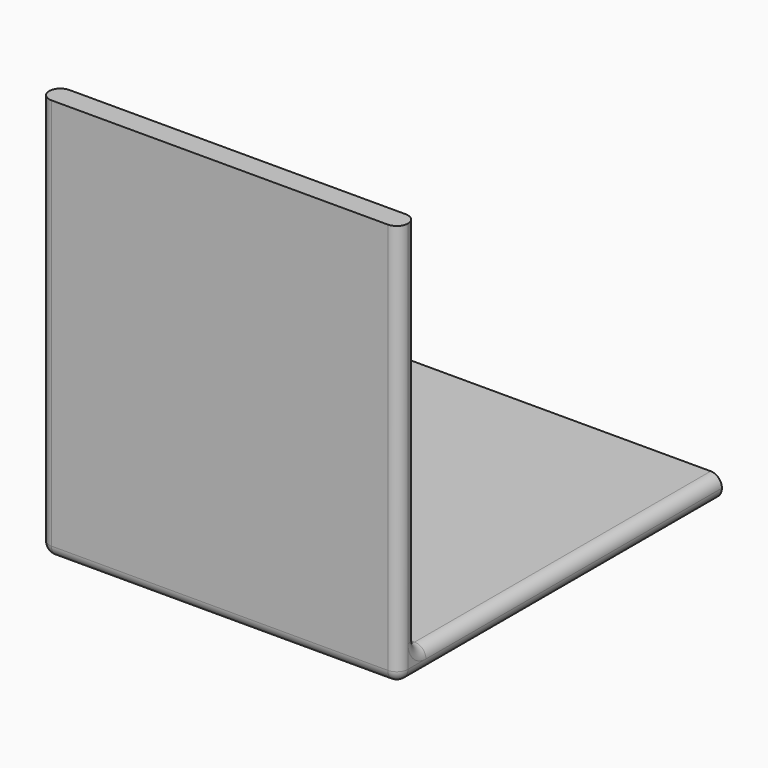
from build123d import *

# Parameters (mm, degrees)
F0_W     = 10
F0_H     = 170
F0_H_2   = 10
F0_W_2   = 170
F1_DEPTH = 160
F2_R     = 4.99999


# Not quite as in the source:
# - a fillet or chamfer is up to 0.001 mm smaller than in the source, because OpenCascade refuses the exact size


with BuildPart() as f1:
    # F0 (on Right) → F1 (new body)
    with BuildSketch(Plane.YZ):
        with Locations((-40.9939204156, 85)):
            Rectangle(F0_W, F0_H)
        with Locations((-40.9939204156, -5)):
            Rectangle(F0_W, F0_H_2)
        with Locations((49.0060795844, -5)):
            Rectangle(F0_W_2, F0_H_2)
    extrude(amount=-F1_DEPTH)

    # F2 (radius 5 in the source; OpenCascade refuses exactly that, so slightly less here)
    f2_edges = [f1.edges().sort_by_distance(p)[0] for p in [
        (0, 49.00608, 0),
        (0, 44.00608, -10),
        (-160, 49.00608, 0),
        (-160, 44.00608, -10),
        (-80, -35.99392, 0),
        (-160, -35.99392, 85),
        (-160, -45.99392, 80),
        (0, -35.99392, 85),
        (0, -45.99392, 80),
        (-80, -45.99392, -10),
    ]]
    fillet(f2_edges, radius=F2_R)


solid = f1.part
